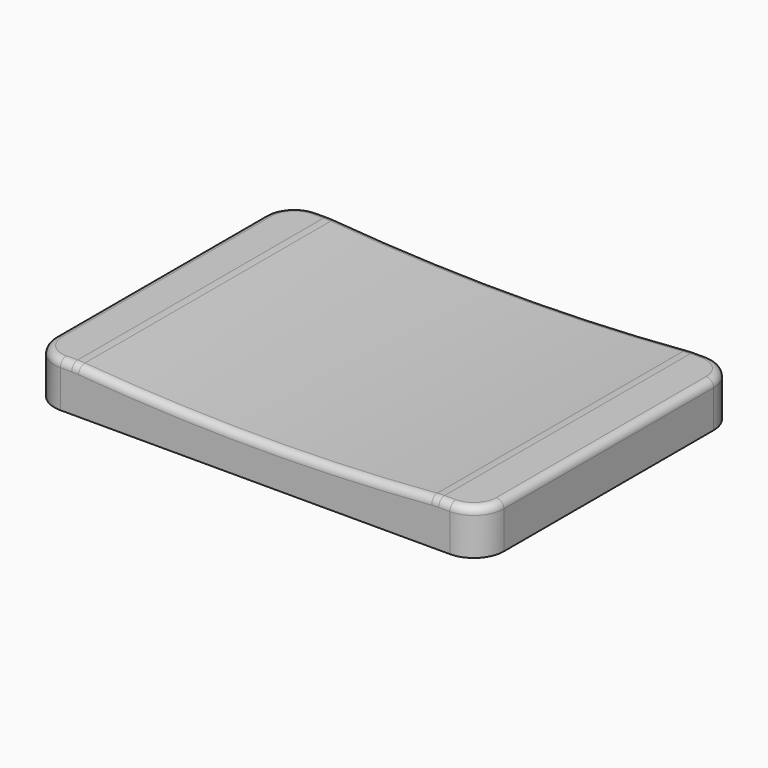
from build123d import *

# Parameters (mm, degrees)
F0_W        = 381
F0_H        = 273.05
F1_DEPTH    = 38.1
F3_DEPTH    = 273.051
F4_T1_DEPTH = 288.7629933337
F5_R        = 25.4
F6_R        = 6.35


# Not quite as in the source:
# - a fillet or chamfer that OpenCascade refuses, or shapes differently, is made with other operations: its cross-section is extruded or revolved along the edge and cut away or added


with BuildPart() as f1:
    # F0 (on Top) → F1 (new body)
    with BuildSketch(Plane.XY):
        Rectangle(F0_W, F0_H)
    extrude(amount=F1_DEPTH)

    # F2 (on face) → F3 (cut, through all)
    with BuildSketch(Plane.XZ.offset(136.525)):
        with BuildLine():
            Line((152.4, 38.1), (-152.4, 38.1))
            ThreePointArc((-152.4, 38.1), (0, 31.75), (152.4, 38.1))
        make_face()
    extrude(amount=-F3_DEPTH, mode=Mode.SUBTRACT)

    # F4: fillet of radius 76.2 on 2 edges, made by hand

    # F4_s2 → F4_t1 (cut)
    with BuildSketch(Plane.XZ.offset(-144.3814966668)):
        with BuildLine():
            ThreePointArc((155.5425986667, 38.1), (152.4343358341, 38.0365792649), (149.3312469729, 37.846422629))
            ThreePointArc((149.3312469729, 37.846422629), (150.8656767636, 37.9725665634), (152.4, 38.1))
            Line((152.4, 38.1), (155.5425986667, 38.1))
        make_face()
        with BuildLine():
            ThreePointArc((-149.3312469729, 37.846422629), (-152.4343358341, 38.0365792649), (-155.5425986667, 38.1))
            Line((-155.5425986667, 38.1), (-152.4, 38.1))
            ThreePointArc((-152.4, 38.1), (-150.8656767636, 37.9725665634), (-149.3312469729, 37.846422629))
        make_face()
    extrude(amount=F4_T1_DEPTH, mode=Mode.SUBTRACT)

    # F5
    f5_edges = [f1.edges().sort_by_distance(p)[0] for p in [
        (-190.5, -136.525, 19.05),
        (190.5, -136.525, 19.05),
        (190.5, 136.525, 19.05),
        (-190.5, 136.525, 19.05),
    ]]
    fillet(f5_edges, radius=F5_R)

    # F6
    f6_edges = [f1.edges().sort_by_distance(p)[0] for p in [
        (160.321299, 136.525, 38.1),
    ]]
    fillet(f6_edges, radius=F6_R)


solid = f1.part
